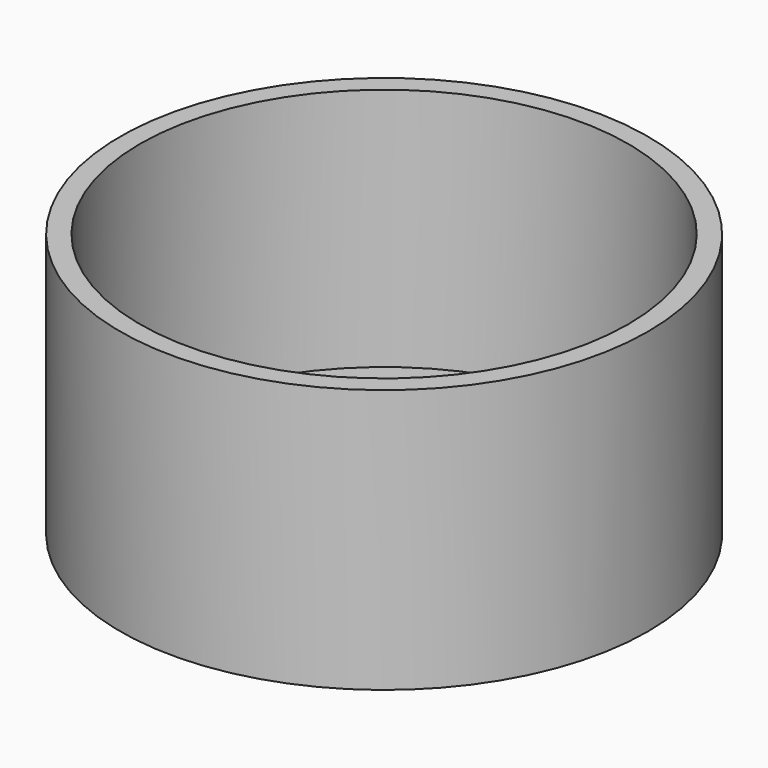
from build123d import *

# Parameters (mm, degrees)
F0_R     = 25.4
F1_DEPTH = 25.4
F4_T     = -1.905


# Not quite as in the source:
# - the program builds the solid bodies; features that only make, move or delete a surface that nothing else refers to are left out


with BuildPart() as f1:
    # F0 (on Top) → F1 (new body)
    with BuildSketch(Plane.XY):
        Circle(F0_R)
    extrude(amount=F1_DEPTH)

    # F4
    f4_openings = [f1.faces().sort_by_distance(p)[0] for p in [
        (0, 0, 25.4),
    ]]
    offset(amount=F4_T, openings=f4_openings)


solid = f1.part
